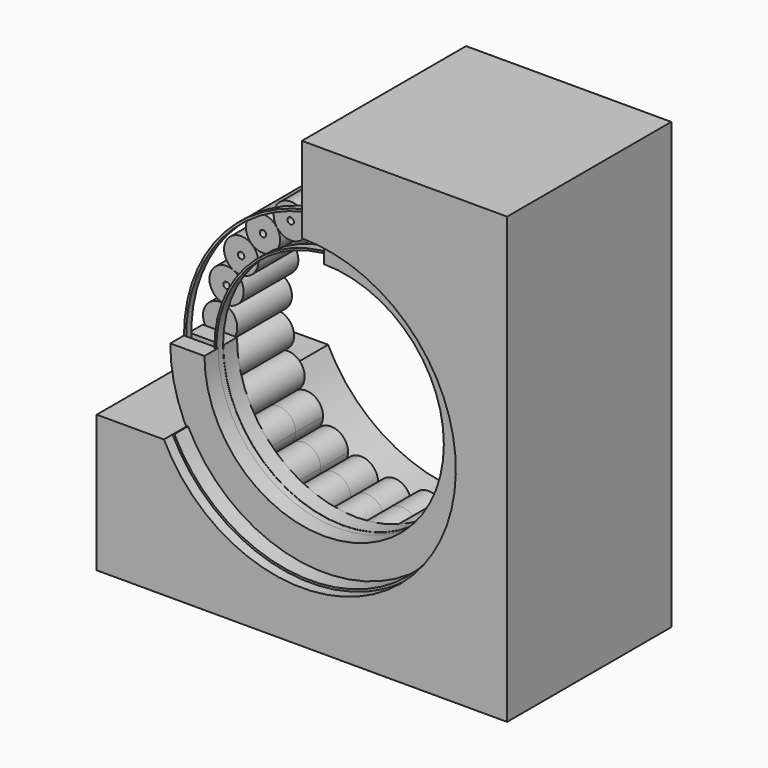
from build123d import *

# Parameters (mm, degrees)
F1_DEPTH  = 304.8
F4_R      = 50.8
F4_R_2    = 9.525
F5_DEPTH  = 101.6
F7_DEPTH  = 50.8
F10_DEPTH = 19.05
F11_DEPTH = 25.4
F13_DEPTH = 50.8
F15_DEPTH = 50.8


# Not quite as in the source:
# - the program builds the solid bodies; features that only make, move or delete a surface that nothing else refers to are left out


with BuildPart() as f1:
    # F0 (on Front) → F1 (new body, symmetric)
    with BuildSketch(Plane.XZ):
        with BuildLine():
            Line((-609.6, -609.6), (0, -609.6))
            Line((0, -609.6), (609.6, -609.6))
            Line((609.6, -609.6), (609.6, 711.9909113884))
            Line((609.6, 711.9909113884), (0, 711.9909113884))
            Line((0, 711.9909113884), (0, 457.2))
            ThreePointArc((0, 457.2), (388.3125515054, -241.3404283235), (-409.9541448106, -202.4090886116))
            Line((-409.9541448106, -202.4090886116), (-609.6, -202.4090886116))
            Line((-609.6, -202.4090886116), (-609.6, -609.6))
        make_face()
    extrude(amount=F1_DEPTH, both=True)

    # F4 (on Front) → F5, piece 9 (join, symmetric)
    with BuildSketch(Plane.XZ):
        with Locations((0, 406.4)):
            Circle(F4_R)
        with Locations((0, 406.4)):
            Circle(F4_R_2, mode=Mode.SUBTRACT)
        with Locations((-313.1365818641, -259.0491094339)):
            Circle(F4_R)
        with Locations((-313.1365818641, -259.0491094339)):
            Circle(F4_R_2, mode=Mode.SUBTRACT)
        with Locations((-238.8759265317, -328.784506514)):
            Circle(F4_R)
        with Locations((-238.8759265317, -328.784506514)):
            Circle(F4_R_2, mode=Mode.SUBTRACT)
        with Locations((-149.6058182111, -377.861163865)):
            Circle(F4_R)
        with Locations((-149.6058182111, -377.861163865)):
            Circle(F4_R_2, mode=Mode.SUBTRACT)
        with Locations((-50.9354261205, -403.1954146142)):
            Circle(F4_R)
        with Locations((-50.9354261205, -403.1954146142)):
            Circle(F4_R_2, mode=Mode.SUBTRACT)
        with Locations((50.9354261205, -403.1954146142)):
            Circle(F4_R)
        with Locations((50.9354261205, -403.1954146142)):
            Circle(F4_R_2, mode=Mode.SUBTRACT)
        with Locations((149.6058182111, -377.861163865)):
            Circle(F4_R)
        with Locations((149.6058182111, -377.861163865)):
            Circle(F4_R_2, mode=Mode.SUBTRACT)
        with Locations((238.8759265317, -328.784506514)):
            Circle(F4_R)
        with Locations((238.8759265317, -328.784506514)):
            Circle(F4_R_2, mode=Mode.SUBTRACT)
        with Locations((313.1365818641, -259.0491094339)):
            Circle(F4_R)
        with Locations((313.1365818641, -259.0491094339)):
            Circle(F4_R_2, mode=Mode.SUBTRACT)
        with Locations((367.7217141222, -173.036704092)):
            Circle(F4_R)
        with Locations((367.7217141222, -173.036704092)):
            Circle(F4_R_2, mode=Mode.SUBTRACT)
        with Locations((399.2015386961, -76.1517662476)):
            Circle(F4_R)
        with Locations((399.2015386961, -76.1517662476)):
            Circle(F4_R_2, mode=Mode.SUBTRACT)
        with Locations((405.5980624332, 25.5180671367)):
            Circle(F4_R)
        with Locations((405.5980624332, 25.5180671367)):
            Circle(F4_R_2, mode=Mode.SUBTRACT)
        with Locations((386.5093682224, 125.584506514)):
            Circle(F4_R)
        with Locations((386.5093682224, 125.584506514)):
            Circle(F4_R_2, mode=Mode.SUBTRACT)
        with Locations((343.134868924, 217.7600094795)):
            Circle(F4_R)
        with Locations((343.134868924, 217.7600094795)):
            Circle(F4_R_2, mode=Mode.SUBTRACT)
        with Locations((278.1999438494, 296.2528501841)):
            Circle(F4_R)
        with Locations((278.1999438494, 296.2528501841)):
            Circle(F4_R_2, mode=Mode.SUBTRACT)
        with Locations((195.7846931549, 356.1310347698)):
            Circle(F4_R)
        with Locations((195.7846931549, 356.1310347698)):
            Circle(F4_R_2, mode=Mode.SUBTRACT)
        with Locations((101.0675701438, 393.6321966827)):
            Circle(F4_R)
        with Locations((101.0675701438, 393.6321966827)):
            Circle(F4_R_2, mode=Mode.SUBTRACT)
    extrude(amount=F5_DEPTH, both=True)


with BuildPart() as f5:
    # F4 (on Front) → F5 (new body, symmetric)
    with BuildSketch(Plane.XZ):
        with Locations((-101.0675701438, 393.6321966827)):
            Circle(F4_R)
        with Locations((-101.0675701438, 393.6321966827)):
            Circle(F4_R_2, mode=Mode.SUBTRACT)
    extrude(amount=F5_DEPTH, both=True)


with BuildPart() as f5b:
    # F4 (on Front) → F5, piece 2 (new body, symmetric)
    with BuildSketch(Plane.XZ):
        with Locations((-195.7846931549, 356.1310347698)):
            Circle(F4_R)
        with Locations((-195.7846931549, 356.1310347698)):
            Circle(F4_R_2, mode=Mode.SUBTRACT)
    extrude(amount=F5_DEPTH, both=True)


with BuildPart() as f5c:
    # F4 (on Front) → F5, piece 3 (new body, symmetric)
    with BuildSketch(Plane.XZ):
        with Locations((-278.1999438494, 296.2528501841)):
            Circle(F4_R)
        with Locations((-278.1999438494, 296.2528501841)):
            Circle(F4_R_2, mode=Mode.SUBTRACT)
    extrude(amount=F5_DEPTH, both=True)


with BuildPart() as f5d:
    # F4 (on Front) → F5, piece 4 (new body, symmetric)
    with BuildSketch(Plane.XZ):
        with Locations((-343.134868924, 217.7600094795)):
            Circle(F4_R)
        with Locations((-343.134868924, 217.7600094795)):
            Circle(F4_R_2, mode=Mode.SUBTRACT)
    extrude(amount=F5_DEPTH, both=True)


with BuildPart() as f5e:
    # F4 (on Front) → F5, piece 5 (new body, symmetric)
    with BuildSketch(Plane.XZ):
        with Locations((-386.5093682224, 125.584506514)):
            Circle(F4_R)
        with Locations((-386.5093682224, 125.584506514)):
            Circle(F4_R_2, mode=Mode.SUBTRACT)
    extrude(amount=F5_DEPTH, both=True)


with BuildPart() as f5f:
    # F4 (on Front) → F5, piece 6 (new body, symmetric)
    with BuildSketch(Plane.XZ):
        with Locations((-405.5980624332, 25.5180671367)):
            Circle(F4_R)
        with Locations((-405.5980624332, 25.5180671367)):
            Circle(F4_R_2, mode=Mode.SUBTRACT)
    extrude(amount=F5_DEPTH, both=True)


with BuildPart() as f5g:
    # F4 (on Front) → F5, piece 7 (new body, symmetric)
    with BuildSketch(Plane.XZ):
        with Locations((-399.2015386961, -76.1517662476)):
            Circle(F4_R)
        with Locations((-399.2015386961, -76.1517662476)):
            Circle(F4_R_2, mode=Mode.SUBTRACT)
    extrude(amount=F5_DEPTH, both=True)


with BuildPart() as f5h:
    # F4 (on Front) → F5, piece 8 (new body, symmetric)
    with BuildSketch(Plane.XZ):
        with Locations((-367.7217141222, -173.036704092)):
            Circle(F4_R)
        with Locations((-367.7217141222, -173.036704092)):
            Circle(F4_R_2, mode=Mode.SUBTRACT)
    extrude(amount=F5_DEPTH, both=True)


with BuildPart() as f7:
    # F6 (on face) → F7 (new body)
    with BuildSketch(Plane.XZ.offset(101.6)):
        with BuildLine():
            ThreePointArc((0, 355.6), (251.4471713899, -251.4471713899), (-355.6, 0))
            Line((-355.6, 0), (-457.2, 0))
            ThreePointArc((-457.2, 0), (323.2892203585, -323.2892203585), (0, 457.2))
            Line((0, 457.2), (0, 355.6))
        make_face()
    extrude(amount=F7_DEPTH)

    # F8 (on face) → F11 (join)
    with BuildSketch(Plane.XZ.offset(152.4)):
        with BuildLine():
            ThreePointArc((201.5214493808, 300.6607855033), (-319.3340657551, -170.3923617663), (361.95, 0))
            ThreePointArc((361.95, 0), (321.9845814381, 165.3291620257), (210.9140457737, 294.1480372115))
            ThreePointArc((210.9140457737, 294.1480372115), (207.2394620386, 291.8139492882), (202.9869810237, 292.7450439544))
            ThreePointArc((202.9869810237, 292.7450439544), (200.6239559094, 296.4010862059), (201.5214493808, 300.6607855033))
        make_face()
        with BuildLine():
            ThreePointArc((356.235, 0), (-315.6061171856, -165.2154775437), (202.9869810237, 292.7450439544))
            ThreePointArc((202.9869810237, 292.7450439544), (315.6061171856, 165.2154775437), (356.235, 0))
        make_face(mode=Mode.SUBTRACT)
        with BuildLine():
            ThreePointArc((202.9869810237, 292.7450439544), (207.2394620386, 291.8139492882), (210.9140457737, 294.1480372115))
            ThreePointArc((210.9140457737, 294.1480372115), (206.2434565954, 297.4414885513), (201.5214493808, 300.6607855033))
            ThreePointArc((201.5214493808, 300.6607855033), (200.6239559094, 296.4010862059), (202.9869810237, 292.7450439544))
        make_face()
        with BuildLine():
            ThreePointArc((201.5214493808, 300.6607855033), (206.2434565954, 297.4414885513), (210.9140457737, 294.1480372115))
            ThreePointArc((210.9140457737, 294.1480372115), (211.6911002215, 295.71394581), (211.9584565954, 297.4414885513))
            ThreePointArc((211.9584565954, 297.4414885513), (207.9279377868, 302.9026009028), (201.5214493808, 300.6607855033))
        make_face()
    extrude(amount=F11_DEPTH)


with BuildPart() as f10:
    # F9 (on face) → F10 (new body)
    with BuildSketch(Plane.XZ.offset(152.4)):
        with BuildLine():
            Line((0, 450.85), (0, 457.2))
            ThreePointArc((0, 457.2), (-323.2892203585, 323.2892203585), (-457.2, 0))
            Line((-457.2, 0), (-450.85, 0))
            ThreePointArc((-450.85, 0), (-318.799092298, 318.799092298), (0, 450.85))
        make_face()
        with BuildLine():
            ThreePointArc((-457.2, 0), (0, -457.2), (457.2, 0))
            ThreePointArc((457.2, 0), (323.2892203585, 323.2892203585), (0, 457.2))
            Line((0, 457.2), (0, 450.85))
            ThreePointArc((0, 450.85), (318.799092298, 318.799092298), (450.85, 0))
            ThreePointArc((450.85, 0), (0, -450.85), (-450.85, 0))
            Line((-450.85, 0), (-457.2, 0))
        make_face()
    extrude(amount=F10_DEPTH)


with BuildPart() as f13:
    # F12 (on face) → F13 (new body)
    with BuildSketch(Plane.XZ.offset(171.45)):
        with BuildLine():
            Line((-355.6, 0), (-457.2, 0))
            ThreePointArc((-457.2, 0), (323.2892203585, -323.2892203585), (0, 457.2))
            Line((0, 457.2), (0, 355.6))
            ThreePointArc((0, 355.6), (251.4471713899, -251.4471713899), (-355.6, 0))
        make_face()
    extrude(amount=F13_DEPTH)


with BuildPart() as f15:
    # F14 (on face) → F15 (new body)
    with BuildSketch(Plane.XZ.offset(222.25)):
        with BuildLine():
            ThreePointArc((0, 450.85), (382.9369948774, -237.9600396165), (-404.2306863553, -199.6578941809))
            Line((-404.2306863553, -199.6578941809), (-409.9240763039, -202.4699771975))
            ThreePointArc((-409.9240763039, -202.4699771975), (388.3304736785, -241.3115894702), (0, 457.2))
            Line((0, 457.2), (0, 450.85))
        make_face()
    extrude(amount=F15_DEPTH)


solid = Compound([f1.part, f5.part, f5b.part, f5c.part, f5d.part, f5e.part, f5f.part, f5g.part, f5h.part, f7.part, f10.part, f13.part, f15.part])
